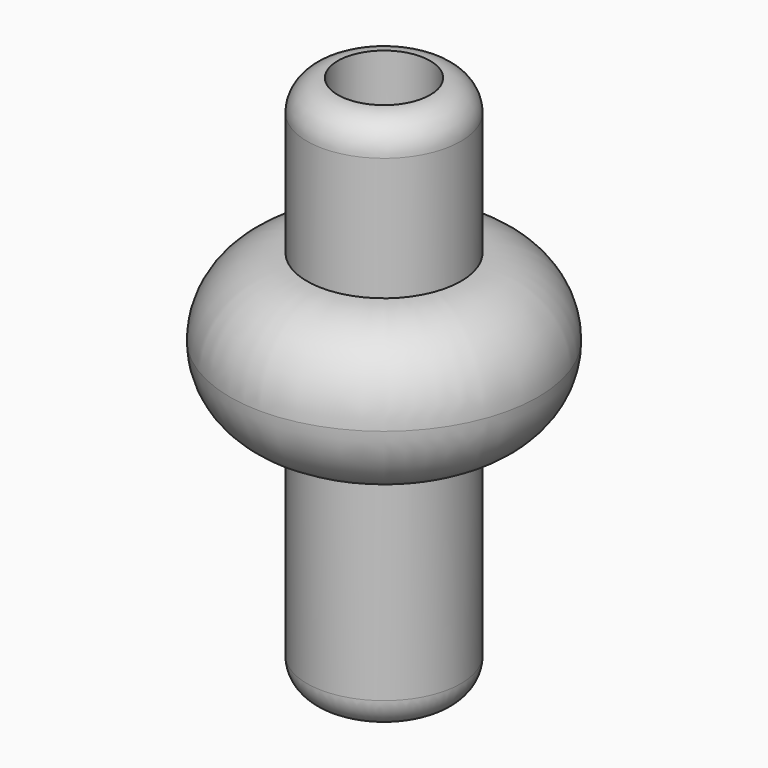
from build123d import *

# Parameters (mm, degrees)
F0_R         = 12.7
F1_DEPTH     = 38.1
F2_R         = 25.4
F2_R_2       = 12.7
F3_DEPTH     = 12.7
F4_R         = 12.69999
F5_R         = 5.07999
F6_T1_DEPTH  = 10.7763073453
F6_T3_DEPTH  = 10.7763073453
F6_T9_DEPTH  = 23.4763073453
F6_S10_R     = 12.7
F6_T11_DEPTH = 14
F6_T15_DEPTH = 23.4763073453
F6_S16_R     = 12.7
F6_T17_DEPTH = 14
F6_T24_DEPTH = 23.4763073453
F6_S25_R     = 12.7
F6_T26_DEPTH = 14
F6_T30_DEPTH = 23.4763073453
F6_S31_R     = 12.7
F6_T32_DEPTH = 14
F6_T39_DEPTH = 23.4763073453
F6_S40_R     = 12.7
F6_T41_DEPTH = 14
F6_T45_DEPTH = 23.4763073453
F6_S46_R     = 12.7
F6_T47_DEPTH = 14
F6_T54_DEPTH = 23.4763073453
F6_S55_R     = 12.7
F6_T56_DEPTH = 14
F6_T60_DEPTH = 23.4763073453
F6_S61_R     = 12.7
F6_T62_DEPTH = 14
F9_R         = 12.7
F9_R_2       = 7.62
F10_DEPTH    = 25.4
F11_R        = 5.07999
F12_DEPTH    = 25.4


# Not quite as in the source:
# - a fillet or chamfer that OpenCascade refuses, or shapes differently, is made with other operations: its cross-section is extruded or revolved along the edge and cut away or added
# - a fillet or chamfer is up to 0.001 mm smaller than in the source, because OpenCascade refuses the exact size


with BuildPart() as f1:
    # F0 (on Top) → F1 (new body)
    with BuildSketch(Plane.XY):
        Circle(F0_R)
        with BuildLine():
            ThreePointArc((5.3881536726, 5.3881536726), (7.0399620377, 2.9160477546), (7.62, 0))
            ThreePointArc((7.62, 0), (7.0399620377, -2.9160477546), (5.3881536726, -5.3881536726))
            ThreePointArc((5.3881536726, -5.3881536726), (0, -7.62), (-5.3881536726, -5.3881536726))
            ThreePointArc((-5.3881536726, -5.3881536726), (-7.62, 0), (-5.3881536726, 5.3881536726))
            ThreePointArc((-5.3881536726, 5.3881536726), (0, 7.62), (5.3881536726, 5.3881536726))
        make_face(mode=Mode.SUBTRACT)
        with BuildLine():
            ThreePointArc((-5.3881536726, -5.3881536726), (0, -7.62), (5.3881536726, -5.3881536726))
            Line((5.3881536726, -5.3881536726), (-5.3881536726, -5.3881536726))
        make_face()
        with BuildLine():
            Line((-5.3881536726, -5.3881536726), (-5.3881536726, 5.3881536726))
            ThreePointArc((-5.3881536726, 5.3881536726), (-7.62, 0), (-5.3881536726, -5.3881536726))
        make_face()
        with BuildLine():
            ThreePointArc((5.3881536726, -5.3881536726), (7.0399620377, -2.9160477546), (7.62, 0))
            ThreePointArc((7.62, 0), (7.0399620377, 2.9160477546), (5.3881536726, 5.3881536726))
            Line((5.3881536726, 5.3881536726), (5.3881536726, -5.3881536726))
        make_face()
        with BuildLine():
            Line((-5.3881536726, 5.3881536726), (5.3881536726, 5.3881536726))
            ThreePointArc((5.3881536726, 5.3881536726), (0, 7.62), (-5.3881536726, 5.3881536726))
        make_face()
    extrude(amount=F1_DEPTH)

    # F5 (radius 5.08 in the source; OpenCascade refuses exactly that, so slightly less here)
    f5_edges = [f1.edges().sort_by_distance(p)[0] for p in [
        (-12.7, 0, 0),
    ]]
    fillet(f5_edges, radius=F5_R)

    # F6: fillet of radius 5.08 on 4 edges, made by hand

    # F6_s2 → F6_t1 (cut)
    with BuildSketch(Plane.XZ.offset(-5.3881536726)):
        with BuildLine():
            ThreePointArc((10.4681536726, 38.1), (6.8760512242, 36.6121024484), (5.3881536726, 33.02))
            Line((5.3881536726, 33.02), (5.3881536726, 38.1))
            Line((5.3881536726, 38.1), (10.4681536726, 38.1))
        make_face()
        with BuildLine():
            ThreePointArc((-10.4681536726, 38.1), (-6.8760512242, 36.6121024484), (-5.3881536726, 33.02))
            Line((-5.3881536726, 33.02), (-5.3881536726, 38.1))
            Line((-5.3881536726, 38.1), (-10.4681536726, 38.1))
        make_face()
    extrude(amount=F6_T1_DEPTH, mode=Mode.SUBTRACT)

    # F6_s4 → F6_t3 (cut)
    with BuildSketch(Plane.YZ.offset(-5.3881536726)):
        with BuildLine():
            ThreePointArc((-10.4681536726, 38.1), (-6.8760512242, 36.6121024484), (-5.3881536726, 33.02))
            Line((-5.3881536726, 33.02), (-5.3881536726, 38.1))
            Line((-5.3881536726, 38.1), (-10.4681536726, 38.1))
        make_face()
        with BuildLine():
            ThreePointArc((10.4681536726, 38.1), (6.8760512242, 36.6121024484), (5.3881536726, 33.02))
            Line((5.3881536726, 33.02), (5.3881536726, 38.1))
            Line((5.3881536726, 38.1), (10.4681536726, 38.1))
        make_face()
    extrude(amount=F6_T3_DEPTH, mode=Mode.SUBTRACT)


with BuildPart() as f3:
    # F2 (on face) → F3 (new body)
    with BuildSketch(Plane.XY.offset(38.1)):
        Circle(F2_R)
        Circle(F2_R_2, mode=Mode.SUBTRACT)
    extrude(amount=F3_DEPTH)

    # F4 (radius 12.7 in the source; OpenCascade refuses exactly that, so slightly less here)
    f4_edges = [f3.edges().sort_by_distance(p)[0] for p in [
        (-25.4, 0, 38.1),
    ]]
    fillet(f4_edges, radius=F4_R)

    # F7: F3 across face


with BuildPart() as f6_tool7:
    # F6_s8 → F6_t9 (new body)
    with BuildSketch(Plane.YZ.offset(-5.3881536726)):
        with BuildLine():
            ThreePointArc((10.4681536726, 38.1), (6.8760512242, 36.6121024484), (5.3881536726, 33.02))
            Line((5.3881536726, 33.02), (5.3881536726, 38.1))
            Line((5.3881536726, 38.1), (10.4681536726, 38.1))
        make_face()
    extrude(amount=F6_T9_DEPTH)

    # F6_s10 → F6_t11 (intersect, symmetric)
    with BuildSketch(Plane.XY.offset(35.6)):
        Circle(F6_S10_R)
    extrude(amount=F6_T11_DEPTH, both=True, mode=Mode.INTERSECT)

    split(bisect_by=Plane.YZ.offset(5.3881536726), keep=Keep.TOP)


with BuildPart() as f6_tool13:
    # F6_s14 → F6_t15 (new body)
    with BuildSketch(Plane.XZ.offset(-18.0881536726)):
        with BuildLine():
            ThreePointArc((10.4681536726, 38.1), (6.8760512242, 36.6121024484), (5.3881536726, 33.02))
            Line((5.3881536726, 33.02), (5.3881536726, 38.1))
            Line((5.3881536726, 38.1), (10.4681536726, 38.1))
        make_face()
    extrude(amount=F6_T15_DEPTH)

    # F6_s16 → F6_t17 (intersect, symmetric)
    with BuildSketch(Plane.XY.offset(35.6)):
        Circle(F6_S16_R)
    extrude(amount=F6_T17_DEPTH, both=True, mode=Mode.INTERSECT)

    split(bisect_by=Plane.XZ.offset(-5.3881536726), keep=Keep.BOTTOM)


with BuildPart() as f6_tool7_1:
    add(f6_tool7.part)

    # F6_t19: intersect F6_tool13
    add(f6_tool13.part, mode=Mode.INTERSECT)


with BuildPart() as f1_1:
    add(f1.part)

    # F6_t5: cut F6_tool7
    add(f6_tool7_1.part, mode=Mode.SUBTRACT)


with BuildPart() as f6_tool22:
    # F6_s23 → F6_t24 (new body)
    with BuildSketch(Plane.YZ.offset(18.0881536726)):
        with BuildLine():
            ThreePointArc((-10.4681536726, 38.1), (-6.8760512242, 36.6121024484), (-5.3881536726, 33.02))
            Line((-5.3881536726, 33.02), (-5.3881536726, 38.1))
            Line((-5.3881536726, 38.1), (-10.4681536726, 38.1))
        make_face()
    extrude(amount=-F6_T24_DEPTH)

    # F6_s25 → F6_t26 (intersect, symmetric)
    with BuildSketch(Plane.XY.offset(35.6)):
        Circle(F6_S25_R)
    extrude(amount=F6_T26_DEPTH, both=True, mode=Mode.INTERSECT)

    split(bisect_by=Plane.YZ.offset(5.3881536726), keep=Keep.TOP)


with BuildPart() as f6_tool28:
    # F6_s29 → F6_t30 (new body)
    with BuildSketch(Plane.XZ.offset(-5.3881536726)):
        with BuildLine():
            ThreePointArc((10.4681536726, 38.1), (6.8760512242, 36.6121024484), (5.3881536726, 33.02))
            Line((5.3881536726, 33.02), (5.3881536726, 38.1))
            Line((5.3881536726, 38.1), (10.4681536726, 38.1))
        make_face()
    extrude(amount=F6_T30_DEPTH)

    # F6_s31 → F6_t32 (intersect, symmetric)
    with BuildSketch(Plane.XY.offset(35.6)):
        Circle(F6_S31_R)
    extrude(amount=F6_T32_DEPTH, both=True, mode=Mode.INTERSECT)

    split(bisect_by=Plane.XZ.offset(5.3881536726), keep=Keep.TOP)


with BuildPart() as f6_tool22_1:
    add(f6_tool22.part)

    # F6_t34: intersect F6_tool28
    add(f6_tool28.part, mode=Mode.INTERSECT)


with BuildPart() as f1_2:
    add(f1_1.part)

    # F6_t20: cut F6_tool22
    add(f6_tool22_1.part, mode=Mode.SUBTRACT)


with BuildPart() as f6_tool37:
    # F6_s38 → F6_t39 (new body)
    with BuildSketch(Plane.YZ.offset(5.3881536726)):
        with BuildLine():
            ThreePointArc((-10.4681536726, 38.1), (-6.8760512242, 36.6121024484), (-5.3881536726, 33.02))
            Line((-5.3881536726, 33.02), (-5.3881536726, 38.1))
            Line((-5.3881536726, 38.1), (-10.4681536726, 38.1))
        make_face()
    extrude(amount=-F6_T39_DEPTH)

    # F6_s40 → F6_t41 (intersect, symmetric)
    with BuildSketch(Plane.XY.offset(35.6)):
        Circle(F6_S40_R)
    extrude(amount=F6_T41_DEPTH, both=True, mode=Mode.INTERSECT)

    split(bisect_by=Plane.YZ.offset(-5.3881536726), keep=Keep.BOTTOM)


with BuildPart() as f6_tool43:
    # F6_s44 → F6_t45 (new body)
    with BuildSketch(Plane.XZ.offset(18.0881536726)):
        with BuildLine():
            ThreePointArc((-10.4681536726, 38.1), (-6.8760512242, 36.6121024484), (-5.3881536726, 33.02))
            Line((-5.3881536726, 33.02), (-5.3881536726, 38.1))
            Line((-5.3881536726, 38.1), (-10.4681536726, 38.1))
        make_face()
    extrude(amount=-F6_T45_DEPTH)

    # F6_s46 → F6_t47 (intersect, symmetric)
    with BuildSketch(Plane.XY.offset(35.6)):
        Circle(F6_S46_R)
    extrude(amount=F6_T47_DEPTH, both=True, mode=Mode.INTERSECT)

    split(bisect_by=Plane.XZ.offset(5.3881536726), keep=Keep.TOP)


with BuildPart() as f6_tool37_1:
    add(f6_tool37.part)

    # F6_t49: intersect F6_tool43
    add(f6_tool43.part, mode=Mode.INTERSECT)


with BuildPart() as f1_3:
    add(f1_2.part)

    # F6_t35: cut F6_tool37
    add(f6_tool37_1.part, mode=Mode.SUBTRACT)


with BuildPart() as f6_tool52:
    # F6_s53 → F6_t54 (new body)
    with BuildSketch(Plane.XZ.offset(5.3881536726)):
        with BuildLine():
            ThreePointArc((-10.4681536726, 38.1), (-6.8760512242, 36.6121024484), (-5.3881536726, 33.02))
            Line((-5.3881536726, 33.02), (-5.3881536726, 38.1))
            Line((-5.3881536726, 38.1), (-10.4681536726, 38.1))
        make_face()
    extrude(amount=-F6_T54_DEPTH)

    # F6_s55 → F6_t56 (intersect, symmetric)
    with BuildSketch(Plane.XY.offset(35.6)):
        Circle(F6_S55_R)
    extrude(amount=F6_T56_DEPTH, both=True, mode=Mode.INTERSECT)

    split(bisect_by=Plane.XZ.offset(-5.3881536726), keep=Keep.BOTTOM)


with BuildPart() as f6_tool58:
    # F6_s59 → F6_t60 (new body)
    with BuildSketch(Plane.YZ.offset(-18.0881536726)):
        with BuildLine():
            ThreePointArc((10.4681536726, 38.1), (6.8760512242, 36.6121024484), (5.3881536726, 33.02))
            Line((5.3881536726, 33.02), (5.3881536726, 38.1))
            Line((5.3881536726, 38.1), (10.4681536726, 38.1))
        make_face()
    extrude(amount=F6_T60_DEPTH)

    # F6_s61 → F6_t62 (intersect, symmetric)
    with BuildSketch(Plane.XY.offset(35.6)):
        Circle(F6_S61_R)
    extrude(amount=F6_T62_DEPTH, both=True, mode=Mode.INTERSECT)

    split(bisect_by=Plane.YZ.offset(-5.3881536726), keep=Keep.BOTTOM)


with BuildPart() as f6_tool52_1:
    add(f6_tool52.part)

    # F6_t64: intersect F6_tool58
    add(f6_tool58.part, mode=Mode.INTERSECT)


with BuildPart() as f1_4:
    add(f1_3.part)

    # F6_t50: cut F6_tool52
    add(f6_tool52_1.part, mode=Mode.SUBTRACT)


with BuildPart() as f3_1:
    add(f3.part)
    add(f3.part.mirror(Plane.XY.offset(50.8)))


with BuildPart() as f10:
    # F9 (on offset) → F10 (new body)
    with BuildSketch(Plane.XY.offset(63.5)):
        Circle(F9_R)
        Circle(F9_R_2, mode=Mode.SUBTRACT)
    extrude(amount=F10_DEPTH)

    # F11 (radius 5.08 in the source; OpenCascade refuses exactly that, so slightly less here)
    f11_edges = [f10.edges().sort_by_distance(p)[0] for p in [
        (-12.7, 0, 88.9),
    ]]
    fillet(f11_edges, radius=F11_R)

    # F9 (on offset) → F12 (join)
    with BuildSketch(Plane.XY.offset(63.5)):
        Circle(F9_R)
        Circle(F9_R_2, mode=Mode.SUBTRACT)
    extrude(amount=-F12_DEPTH)


solid = Compound([f1_4.part, f3_1.part, f10.part])
